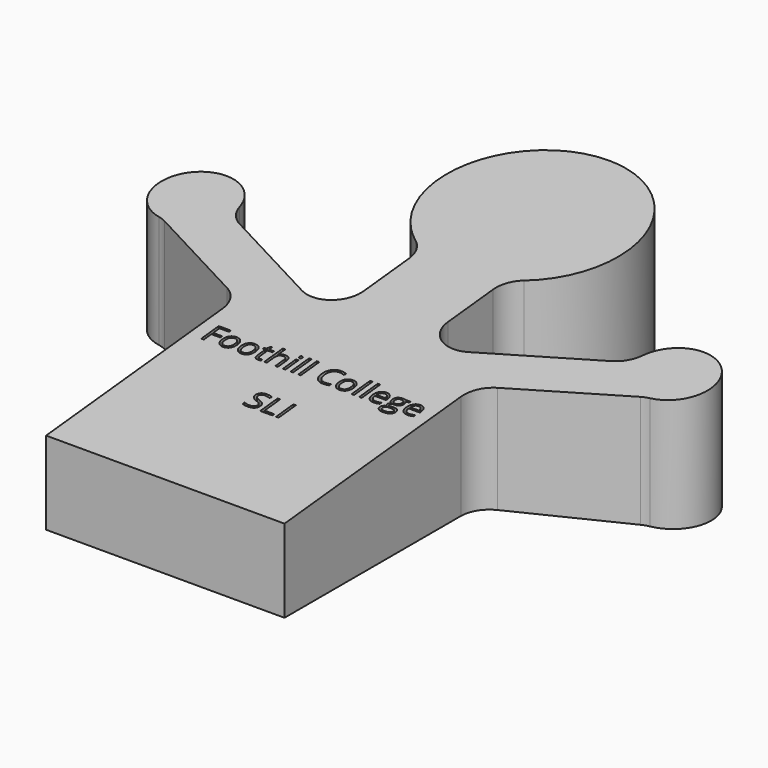
from build123d import *

# Parameters (mm, degrees)
F3_REACH     = 96.6769810013
F5_TEXT_SIZE = 3.1944444444
F6_DEPTH     = 25


# Not quite as in the source:
# - Text() gives the source's letters only with a copy of the font that has no kerning and outlines rounded to 1/6400 em; it was checked with that copy


with BuildPart() as f3:
    f3_end = Plane(origin=(0, -1.0509781927, 10.4805876953), x_dir=(0, 0.9950097103, 0.0997781362), z_dir=(0, -0.0997781362, 0.9950097103))
    # F2 (on Top) → F3 (new body, up to a plane its end follows)
    with BuildSketch(Plane.XY):
        with BuildLine():
            ThreePointArc((5.6970879577, 21.0519185097), (9.5442302804, 32.2549565592), (0, 39.2703848388))
            ThreePointArc((0, 39.2703848388), (-9.5442302804, 32.2549565592), (-5.6970879577, 21.0519185097))
            ThreePointArc((-5.6970879577, 21.0519185097), (-4.7484540885, 19.9778923259), (-4.406214345, 18.5863786109))
            Line((-4.406214345, 18.5863786109), (-4.406214345, 12.6560893326))
            ThreePointArc((-4.406214345, 12.6560893326), (-5.8176375882, 10.1112074321), (-8.7238302702, 9.9609291753))
            Line((-8.7238302702, 9.9609291753), (-19.5044708995, 15.2313928762))
            ThreePointArc((-19.5044708995, 15.2313928762), (-20.5442950135, 16.0711618453), (-21.1161813957, 17.2792148554))
            ThreePointArc((-21.1161813957, 17.2792148554), (-27.9017908151, 19.1921586374), (-25.7412017699, 12.4812940072))
            ThreePointArc((-25.7412017699, 12.4812940072), (-25.3433361251, 12.3800091341), (-24.963024704, 12.2253517067))
            Line((-24.963024704, 12.2253517067), (-14.1823840748, 6.9548880057))
            ThreePointArc((-14.1823840748, 6.9548880057), (-12.9551180994, 5.8483046052), (-12.5, 4.2597278484))
            Line((-12.5, 4.2597278484), (-12.5, -18.8675996833))
            Line((-12.5, -18.8675996833), (0, -18.8675996833))
            Line((0, -18.8675996833), (12.5, -18.8675996833))
            Line((12.5, -18.8675996833), (12.5, 4.2597278484))
            ThreePointArc((12.5, 4.2597278484), (12.9551180994, 5.8483046052), (14.1823840748, 6.9548880057))
            Line((14.1823840748, 6.9548880057), (24.963024704, 12.2253517067))
            ThreePointArc((24.963024704, 12.2253517067), (25.3433361251, 12.3800091341), (25.7412017699, 12.4812940072))
            ThreePointArc((25.7412017699, 12.4812940072), (27.9017908151, 19.1921586374), (21.1161813957, 17.2792148554))
            ThreePointArc((21.1161813957, 17.2792148554), (20.5442950135, 16.0711618453), (19.5044708995, 15.2313928762))
            Line((19.5044708995, 15.2313928762), (8.7238302702, 9.9609291753))
            ThreePointArc((8.7238302702, 9.9609291753), (5.8176375882, 10.1112074321), (4.406214345, 12.6560893326))
            Line((4.406214345, 12.6560893326), (4.406214345, 18.5863786109))
            ThreePointArc((4.406214345, 18.5863786109), (4.7484540885, 19.9778923259), (5.6970879577, 21.0519185097))
        make_face()
    f3_long = extrude(amount=F3_REACH, mode=Mode.PRIVATE)
    add(split(f3_long, bisect_by=f3_end, keep=Keep.BOTTOM, mode=Mode.PRIVATE))

    # F5 (on offset) → F6 (cut)
    with BuildSketch(Plane.XY.offset(8)):
        with Locations((-11.3931857639, -0.2920310483)):
            Text('Foothill College', F5_TEXT_SIZE, font='Open Sans', text_align=(TextAlign.LEFT, TextAlign.BOTTOM))
        with Locations((-2.0986002604, -6.383448513)):
            Text('SLI', F5_TEXT_SIZE, font='Open Sans', text_align=(TextAlign.LEFT, TextAlign.BOTTOM))
    extrude(amount=F6_DEPTH, mode=Mode.SUBTRACT)


solid = f3.part
